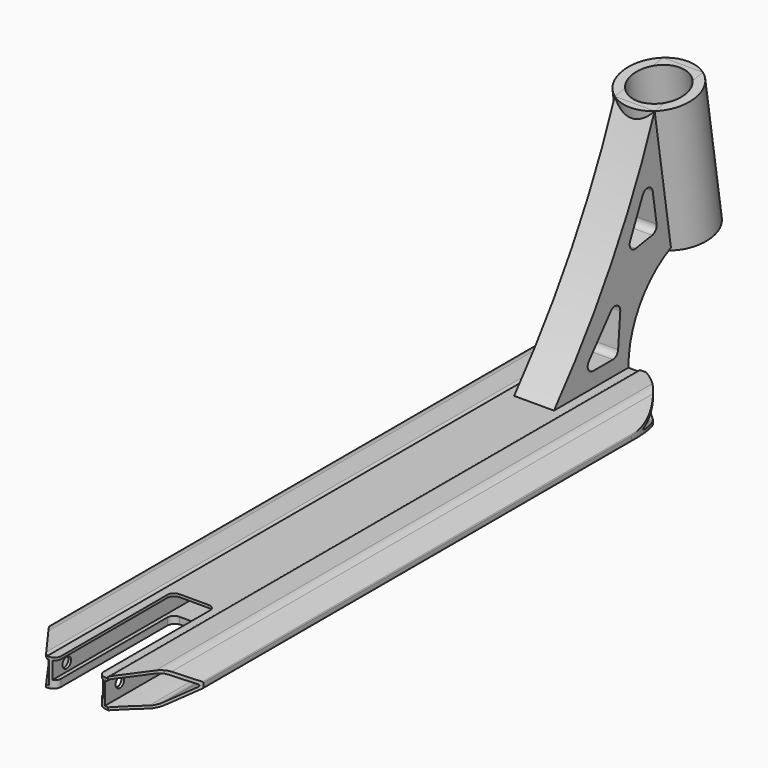
from build123d import *

# Parameters (mm, degrees)
F1_DEPTH    = 250
F2_W        = 38
F2_H        = 13
F3_DEPTH    = 250
F4_T1_DEPTH = 509.3674969976
F5_R        = 9
F6_R        = 1
F8_DEPTH    = 500.001
F10_DEPTH   = 26.9812669128
F11_W       = 10.5
F11_H       = 54
F12_DEPTH   = 26.9812670128
F13_R       = 4.99999
F15_DEPTH   = 15
F16_R       = 27.4590604355
F17_DEPTH   = 100
F19_D       = 40
F21_D       = 8
F23_DEPTH   = 72.5010001
F24_R       = 5


# Not quite as in the source:
# - a fillet or chamfer that OpenCascade refuses, or shapes differently, is made with other operations: its cross-section is extruded or revolved along the edge and cut away or added
# - a fillet or chamfer is up to 0.001 mm smaller than in the source, because OpenCascade refuses the exact size


with BuildPart() as f1:
    # F0 (on Front) → F1 (new body, symmetric)
    with BuildSketch(Plane.XZ):
        with BuildLine():
            Line((22.5, 25.6802669128), (0, 25.6802669128))
            Line((0, 25.6802669128), (-22.5, 25.6802669128))
            Line((-22.5, 25.6802669128), (-22.5, 26.9802669128))
            Line((-22.5, 26.9802669128), (-43.5443276317, 26.9802669128))
            Line((-43.5443276317, 26.9802669128), (-57.5, 15.2700673757))
            Line((-57.5, 15.2700673757), (-57.5, 11.2700673757))
            Line((-57.5, 11.2700673757), (-40.8899783638, 1.6802669128))
            ThreePointArc((-40.8899783638, 1.6802669128), (0, 5.9048607214), (40.8899783638, 1.6802669128))
            Line((40.8899783638, 1.6802669128), (57.5, 11.2700673757))
            Line((57.5, 11.2700673757), (57.5, 15.2700673757))
            Line((57.5, 15.2700673757), (43.5443276317, 26.9802669128))
            Line((43.5443276317, 26.9802669128), (22.5, 26.9802669128))
            Line((22.5, 26.9802669128), (22.5, 25.6802669128))
        make_face()
    extrude(amount=F1_DEPTH, both=True)

    # F2 (on Front) → F3 (cut, symmetric)
    with BuildSketch(Plane.XZ):
        with Locations((0, 17.1802669128)):
            Rectangle(F2_W, F2_H)
    extrude(amount=F3_DEPTH, both=True, mode=Mode.SUBTRACT)

    # F4: fillet of radius 2 on 2 edges, made by hand

    # F4_s2 → F4_t1 (cut)
    with BuildSketch(Plane.XZ.offset(-254.6837484988)):
        with BuildLine():
            ThreePointArc((-24.3734993995, 26.9802669128), (-23.2333239744, 26.6234345853), (-22.5, 25.6802669128))
            Line((-22.5, 25.6802669128), (-22.5, 26.9802669128))
            Line((-22.5, 26.9802669128), (-24.3734993995, 26.9802669128))
        make_face()
        with BuildLine():
            ThreePointArc((24.3734993995, 26.9802669128), (23.2333239744, 26.6234345853), (22.5, 25.6802669128))
            Line((22.5, 25.6802669128), (22.5, 26.9802669128))
            Line((22.5, 26.9802669128), (24.3734993995, 26.9802669128))
        make_face()
    extrude(amount=F4_T1_DEPTH, mode=Mode.SUBTRACT)

    # F5
    f5_edges = [f1.edges().sort_by_distance(p)[0] for p in [
        (43.544328, 0, 26.980267),
        (-43.544328, 0, 26.980267),
        (-40.889978, 0, 1.680267),
        (40.889978, 0, 1.680267),
    ]]
    fillet(f5_edges, radius=F5_R)

    # F6
    f6_edges = [f1.edges().sort_by_distance(p)[0] for p in [
        (57.5, 0, 15.270067),
        (57.5, 0, 11.270067),
        (-57.5, 0, 15.270067),
        (-57.5, 0, 11.270067),
    ]]
    fillet(f6_edges, radius=F6_R)

    # F7 (on face) → F8 (cut, through all)
    with BuildSketch(Plane.XZ.offset(250)):
        with BuildLine():
            ThreePointArc((-55.7563117574, 14.1223809582), (-56.1097188459, 13.2691807724), (-55.6135241478, 12.4903111113))
            Line((-55.6135241478, 12.4903111113), (-42.8286897057, 5.1089835047))
            ThreePointArc((-42.8286897057, 5.1089835047), (-40.4932803063, 4.2687176528), (-38.0114608639, 4.2962134638))
            ThreePointArc((-38.0114608639, 4.2962134638), (-29.5324956629, 5.7343673012), (-21, 6.8103111203))
            Line((-21, 6.8103111203), (-21, 23.6802669128))
            Line((-21, 23.6802669128), (-22.5, 23.6802669128))
            ThreePointArc((-22.5, 23.6802669128), (-23.2333239744, 24.6234345853), (-24.3734993995, 24.9802669128))
            Line((-24.3734993995, 24.9802669128), (-40.2685955233, 24.9802669128))
            ThreePointArc((-40.2685955233, 24.9802669128), (-42.6627365266, 24.5581152583), (-44.7681087911, 23.3425780146))
            Line((-44.7681087911, 23.3425780146), (-55.7563117574, 14.1223809582))
        make_face()
        with BuildLine():
            ThreePointArc((44.7681087911, 23.3425780146), (42.6627365266, 24.5581152583), (40.2685955233, 24.9802669128))
            Line((40.2685955233, 24.9802669128), (24.3734993995, 24.9802669128))
            ThreePointArc((24.3734993995, 24.9802669128), (23.2333239744, 24.6234345853), (22.5, 23.6802669128))
            Line((22.5, 23.6802669128), (21, 23.6802669128))
            Line((21, 23.6802669128), (21, 6.8103111203))
            ThreePointArc((21, 6.8103111203), (29.5324956629, 5.7343673012), (38.0114608639, 4.2962134638))
            ThreePointArc((38.0114608639, 4.2962134638), (40.4932803063, 4.2687176528), (42.8286897057, 5.1089835047))
            Line((42.8286897057, 5.1089835047), (55.6135241478, 12.4903111113))
            ThreePointArc((55.6135241478, 12.4903111113), (56.1097188459, 13.2691807724), (55.7563117574, 14.1223809582))
            Line((55.7563117574, 14.1223809582), (44.7681087911, 23.3425780146))
        make_face()
    extrude(amount=-F8_DEPTH, mode=Mode.SUBTRACT)

    # F9 (on Top) → F10 (cut, through all)
    with BuildSketch(Plane.XY):
        with BuildLine():
            ThreePointArc((-57.5, 200), (0, 257.5), (57.5, 200))
            Line((57.5, 200), (57.5, 280))
            Line((57.5, 280), (-57.5, 280))
            Line((-57.5, 280), (-57.5, 200))
        make_face()
    extrude(amount=F10_DEPTH, mode=Mode.SUBTRACT)

    # F11 (on Top) → F12 (cut, through all)
    with BuildSketch(Plane.XY):
        Polygon((-23.3525011837, -250), (-57.5, -203), (-57.5, -257), (-57.5, -303), (57.5, -303), (57.5, -257), (57.5, -203), (23.3525011837, -250), (16, -250), (16, -140), (-16, -140), (-16, -250), align=None)
        with Locations((-62.75, -230)):
            Rectangle(F11_W, F11_H)
        with Locations((62.75, -230)):
            Rectangle(F11_W, F11_H)
    extrude(amount=F12_DEPTH, mode=Mode.SUBTRACT)

    # F13 (radius 5 in the source; OpenCascade refuses exactly that, so slightly less here)
    f13_edges = [f1.edges().sort_by_distance(p)[0] for p in [
        (-16, -250, 24.680267),
        (-16, -140, 24.680267),
        (-16, -140, 7.97205),
        (16, -250, 24.680267),
        (16, -140, 7.97205),
        (16, -140, 24.680267),
    ]]
    fillet(f13_edges, radius=F13_R)

    # F14 (on Right) → F15 (join, symmetric)
    with BuildSketch(Plane.YZ):
        with BuildLine():
            Line((180, 25.6802669128), (250, 25.6802669128))
            ThreePointArc((250, 25.6802669128), (260.8542924596, 63.1206899813), (290.0510079871, 88.9499901413))
            Line((290.0510079871, 88.9499901413), (290.3738837422, 86.9114328533))
            Line((290.3738837422, 86.9114328533), (335.8075474096, 94.1074182451))
            Line((335.8075474096, 94.1074182451), (320.1641009056, 192.8762523046))
            Line((320.1641009056, 192.8762523046), (274.7304372382, 185.6802669128))
            ThreePointArc((274.7304372382, 185.6802669128), (234.1756922296, 101.6480222695), (180, 25.6802669128))
        make_face()
    extrude(amount=F15_DEPTH, both=True)

    # F16 (on face) → F17 (join, through all)
    with BuildSketch(Plane(origin=(0, -21.966046659, 138.6881603645), x_dir=(1, 0, 0), z_dir=(0, -0.156434465, 0.9876883406))):
        with Locations((0, 323.3948428898)):
            Circle(F16_R)
    extrude(amount=-F17_DEPTH)

    # F19 (through all)
    with Locations(Plane(origin=(0, -21.966046659, 138.6881603645), x_dir=(1, 0, 0), z_dir=(0, -0.156434465, 0.9876883406))):
        with Locations((0, 323.3948428898)):
            Hole(F19_D / 2)

    # F21 (through all)
    with Locations(Plane.YZ.offset(21)):
        with Locations((-236, 16.8103111203)):
            Hole(F21_D / 2)

    # F22 (on face) → F23 (cut, through all)
    with BuildSketch(Plane.YZ.offset(15)):
        Polygon((243.6360210934, 81.8331302618), (206, 36.9802669128), (240, 36.9802669128), align=None)
        Polygon((277.3683110355, 105.1008550147), (270.3287601087, 149.5468303415), (247.7376608176, 100.4078210635), align=None)
    extrude(amount=-F23_DEPTH, mode=Mode.SUBTRACT)

    # F24
    f24_edges = [f1.edges().sort_by_distance(p)[0] for p in [
        (0, 270.32876, 149.54683),
        (0, 240, 36.980267),
        (0, 277.368311, 105.100855),
        (0, 243.636021, 81.83313),
        (0, 247.737661, 100.407821),
        (0, 206, 36.980267),
    ]]
    fillet(f24_edges, radius=F24_R)


solid = f1.part
